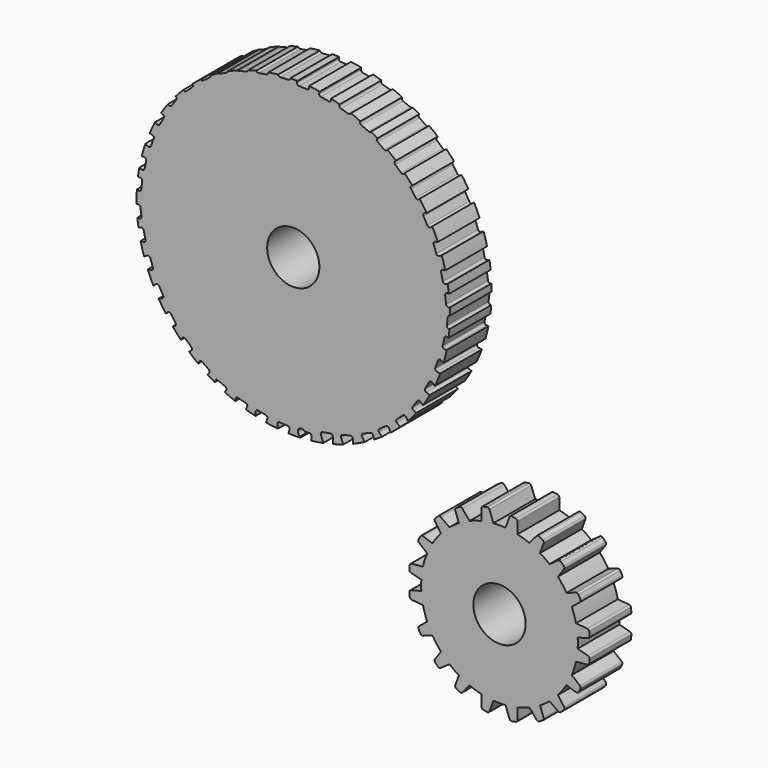
from build123d import *

# Parameters (mm, degrees)
F0_R     = 6.35
F1_DEPTH = 12.7
F2_R     = 6.35
F3_DEPTH = 6.35
F4_DEPTH = 12.7


# Not quite as in the source:
# - a feature names something its author has since deleted; it is built from what else it names


with BuildPart() as f1:
    # F0 (on Front) → F1 (new body)
    with BuildSketch(Plane.XZ):
        with BuildLine():
            ThreePointArc((10.9997188912, 27.5581906646), (10.9998077873, 27.6057086098), (10.9998374194, 27.6532266289))
            ThreePointArc((10.9998374194, 27.6532266289), (10.9910152614, 28.4730867424), (10.9645528732, 29.2925671742))
            Line((10.9645528732, 29.2925671742), (10.7348382856, 29.2197734001))
            ThreePointArc((10.7348382856, 29.2197734001), (10.3090510106, 29.2752036537), (10.0778222636, 29.6370055099))
            Line((10.0778222636, 29.6370055099), (9.8220033848, 31.5586845929))
            ThreePointArc((9.8220033848, 31.5586845929), (9.9505287127, 31.96837784), (10.3469864363, 32.1332674697))
            Line((10.3469864363, 32.1332674697), (10.7374728979, 32.1167836625))
            ThreePointArc((10.7374728979, 32.1167836625), (10.6025380467, 33.1410645829), (10.4398806598, 34.1613103339))
            Line((10.4398806598, 34.1613103339), (9.9591086943, 33.9605689489))
            ThreePointArc((9.9591086943, 33.9605689489), (9.5300858292, 33.9780817406), (9.2677308241, 34.3179893279))
            Line((9.2677308241, 34.3179893279), (8.8427687035, 36.2094704916))
            ThreePointArc((8.8427687035, 36.2094704916), (8.9345144752, 36.6289344709), (9.314815571, 36.8282793809))
            Line((9.314815571, 36.8282793809), (9.8721533535, 36.8541969291))
            ThreePointArc((9.8721533535, 36.8541969291), (9.4699352014, 38.3414420184), (9.0079175064, 39.811209703))
            Line((9.0079175064, 39.811209703), (8.4039697241, 39.4688653608))
            ThreePointArc((8.4039697241, 39.4688653608), (7.9759406786, 39.4348293087), (7.674735783, 39.7408406278))
            Line((7.674735783, 39.7408406278), (7.0261247489, 41.5677499095))
            ThreePointArc((7.0261247489, 41.5677499095), (7.0669322446, 41.9951865303), (7.4205982455, 42.2386771389))
            Line((7.4205982455, 42.2386771389), (8.0532126762, 42.3450681763))
            ThreePointArc((8.0532126762, 42.3450681763), (7.4021635025, 43.8148940816), (6.6896909802, 45.2559479055))
            Line((6.6896909802, 45.2559479055), (6.306212971, 44.9339528718))
            ThreePointArc((6.306212971, 44.9339528718), (5.8915008094, 44.8226823023), (5.539690769, 45.0688469058))
            Line((5.539690769, 45.0688469058), (4.5698129336, 46.7474268953))
            ThreePointArc((4.5698129336, 46.7474268953), (4.5322468252, 47.1751605789), (4.8357628076, 47.4788797996))
            Line((4.8357628076, 47.4788797996), (5.3257876329, 47.6574200081))
            ThreePointArc((5.3257876329, 47.6574200081), (4.5033634367, 48.9329621365), (3.63079132, 50.1747379539))
            Line((3.63079132, 50.1747379539), (3.4411244827, 49.9830087806))
            ThreePointArc((3.4411244827, 49.9830087806), (3.0384391107, 49.8339725172), (2.6654295416, 50.0466487452))
            Line((2.6654295416, 50.0466487452), (1.5449052905, 51.6286472279))
            ThreePointArc((1.5449052905, 51.6286472279), (1.4680588038, 52.0510947798), (1.742276434, 52.381506656))
            Line((1.742276434, 52.381506656), (1.8437067996, 52.4294738286))
            ThreePointArc((1.8437067996, 52.4294738286), (0.9185212718, 53.4711149077), (-0.044128746, 54.4782342364))
            Line((-0.044128746, 54.4782342364), (-0.1099293962, 54.3743183929))
            ThreePointArc((-0.1099293962, 54.3743183929), (-0.4714291441, 54.1426176184), (-0.8812897937, 54.2706081044))
            Line((-0.8812897937, 54.2706081044), (-2.3141954623, 55.5763933629))
            ThreePointArc((-2.3141954623, 55.5763933629), (-2.479602409, 55.9726355346), (-2.2823848312, 56.3540441653))
            Line((-2.2823848312, 56.3540441653), (-2.155429431, 56.4520163273))
            ThreePointArc((-2.155429431, 56.4520163274), (-3.1700394132, 57.3004727944), (-4.2134872008, 58.1132018433))
            Line((-4.2134872008, 58.1132018433), (-4.2235525545, 58.0920996826))
            ThreePointArc((-4.2235525545, 58.0920996826), (-4.5548743062, 57.8189821009), (-4.9770640288, 57.8972326901))
            Line((-4.9770640288, 57.8972326901), (-6.5553283188, 59.0230104781))
            ThreePointArc((-6.5553283188, 59.0230104781), (-6.765991691, 59.3879047844), (-6.6288005117, 59.7862833625))
            ThreePointArc((-6.6288005117, 59.7862833625), (-7.395295474, 60.2619403771), (-8.1728368701, 60.7193171364))
            ThreePointArc((-8.1728368701, 60.7193171364), (-8.4440936015, 60.5462785431), (-8.7648986851, 60.570909163))
            Line((-8.7648986851, 60.570909163), (-10.5513587328, 61.3238064301))
            ThreePointArc((-10.5513587328, 61.3238064301), (-10.8394888709, 61.6421589707), (-10.7808231589, 62.0675125305))
            Line((-10.7808231589, 62.0675125305), (-10.7740288476, 62.0780339244))
            ThreePointArc((-10.7740288476, 62.0780339244), (-11.9114103089, 62.5947750266), (-13.0651215331, 63.0739496988))
            ThreePointArc((-13.0651215331, 63.0739496988), (-13.308737144, 62.780369269), (-13.687996631, 62.7391348639))
            Line((-13.687996631, 62.7391348639), (-15.5529276076, 63.2685933129))
            ThreePointArc((-15.5529276076, 63.2685933129), (-15.8777243682, 63.5494391441), (-15.8713593131, 63.9787721183))
            Line((-15.8713593131, 63.9787721183), (-15.8367193146, 64.050271094))
            ThreePointArc((-15.8367193146, 64.050271094), (-16.8664088252, 64.3530942591), (-17.9042195936, 64.6267933027))
            Line((-17.9042195936, 64.6267933027), (-17.9048293367, 64.3664165893))
            ThreePointArc((-17.9048293367, 64.3664165893), (-18.0872040332, 63.9776920253), (-18.5022125206, 63.8675318148))
            Line((-18.5022125206, 63.8675318148), (-20.4105987179, 64.2086416483))
            ThreePointArc((-20.4105987179, 64.2086416483), (-20.7617486486, 64.4557469755), (-20.7981698105, 64.8835796713))
            Line((-20.7981698105, 64.8835796713), (-20.6791346872, 65.2082582597))
            ThreePointArc((-20.6791346872, 65.2082582597), (-21.9733949544, 65.4067198938), (-23.2737104471, 65.5605908748))
            Line((-23.2737104471, 65.5605908748), (-23.236864005, 65.2838050588))
            ThreePointArc((-23.236864005, 65.2838050588), (-23.3653893328, 64.8741118118), (-23.7618470564, 64.709222182))
            Line((-23.7618470564, 64.709222182), (-25.6987539983, 64.7909858376))
            ThreePointArc((-25.6987539983, 64.7909858376), (-26.0799048953, 64.9887010627), (-26.1734453199, 65.4077684864))
            Line((-26.1734453199, 65.4077684864), (-26.1002719199, 65.740103879))
            ThreePointArc((-26.1002719199, 65.740103879), (-26.9648411973, 65.7529863148), (-27.8294801715, 65.7462456199))
            ThreePointArc((-27.8294801715, 65.7462456199), (-27.9804758504, 65.4141090568), (-28.3151593807, 65.2688461018))
            Line((-28.3151593807, 65.2688461018), (-30.2520663226, 65.1870824461))
            ThreePointArc((-30.2520663226, 65.1870824461), (-30.579618702, 65.2892290657), (-30.767521052, 65.5763130255))
            ThreePointArc((-30.767521052, 65.5763130255), (-31.9815332506, 65.4392322445), (-33.190526184, 65.2632980351))
            ThreePointArc((-33.190526184, 65.2632980351), (-33.2795908388, 64.890932176), (-33.603314661, 64.6865019124))
            Line((-33.603314661, 64.6865019124), (-35.5117008584, 64.3453920789))
            ThreePointArc((-35.5117008584, 64.3453920789), (-35.858172076, 64.4073221349), (-36.0812348157, 64.6795732149))
            ThreePointArc((-36.0812348157, 64.6795732149), (-37.0957600333, 64.4186727919), (-38.1027291762, 64.1299798878))
            ThreePointArc((-38.1027291762, 64.1299798878), (-38.2284934828, 63.8883687789), (-38.4609857713, 63.746453577))
            Line((-38.4609857713, 63.746453577), (-40.325916748, 63.2169951281))
            ThreePointArc((-40.325916748, 63.2169951281), (-40.5089917117, 63.1996208677), (-40.6862566858, 63.2485640618))
            ThreePointArc((-40.6862566858, 63.2485640618), (-41.9303127886, 62.7484776582), (-43.1560023326, 62.2049271639))
            ThreePointArc((-43.1560023326, 62.2049271639), (-43.2554297219, 61.9623619367), (-43.4625546462, 61.8016666943))
            Line((-43.4625546462, 61.8016666943), (-45.2490146938, 61.0487694271))
            ThreePointArc((-45.2490146938, 61.0487694271), (-45.375143841, 61.0139029847), (-45.5059949449, 61.0124132943))
            ThreePointArc((-45.5059949449, 61.0124132943), (-46.3852858073, 60.5119244444), (-47.2509772507, 59.9882644073))
            ThreePointArc((-47.2509772507, 59.9882644073), (-47.2862171184, 59.7153623746), (-47.4585850602, 59.5008707422))
            Line((-47.4585850602, 59.5008707422), (-49.0368493501, 58.3750929543))
            ThreePointArc((-49.0368493501, 58.3750929543), (-49.3340936045, 58.280667011), (-49.6304916926, 58.3777163742))
            ThreePointArc((-49.6304916926, 58.3777163742), (-50.6630403611, 57.5931797134), (-51.6682920146, 56.7739583524))
            ThreePointArc((-51.6682920146, 56.7739583524), (-51.5343700759, 56.4075721833), (-51.6997179166, 56.0542536271))
            Line((-51.6997179166, 56.0542536271), (-53.1326235853, 54.7484683686))
            ThreePointArc((-53.1326235853, 54.7484683686), (-53.4988929438, 54.6165196483), (-53.8510076529, 54.7825887283))
            ThreePointArc((-53.8510076529, 54.7825887283), (-54.7920642825, 53.8213098628), (-55.6985988975, 52.8274086459))
            ThreePointArc((-55.6985988975, 52.8274086459), (-55.4746545299, 52.4968286533), (-55.5588186695, 52.1065074921))
            Line((-55.5588186695, 52.1065074921), (-56.6793429206, 50.5245090093))
            ThreePointArc((-56.6793429206, 50.5245090093), (-57.0523524897, 50.3118327813), (-57.4550378616, 50.4608690448))
            Line((-57.4550378616, 50.4608690448), (-57.5485150255, 50.5553626295))
            ThreePointArc((-57.5485150255, 50.5553626295), (-58.4221627735, 49.3452137189), (-59.2477420524, 48.1017750886))
            Line((-59.2477420524, 48.1017750886), (-58.8496761866, 47.9567400637))
            ThreePointArc((-58.8496761866, 47.9567400637), (-58.5461602041, 47.6530208431), (-58.5837263125, 47.2252871595))
            Line((-58.5837263125, 47.2252871595), (-59.5536041479, 45.5467071699))
            ThreePointArc((-59.5536041479, 45.5467071699), (-59.9054141884, 45.3005425665), (-60.32012635, 45.411813136))
            Line((-60.32012635, 45.411813136), (-60.6575622622, 45.6951479957))
            ThreePointArc((-60.6575622622, 45.6951479957), (-61.3845046078, 44.2723087866), (-62.0511517876, 42.8202419401))
            Line((-62.0511517876, 42.8202419401), (-61.4345116244, 42.716537403))
            ThreePointArc((-61.4345116244, 42.716537403), (-61.0808456236, 42.4730467945), (-61.0400381279, 42.0456101736))
            Line((-61.0400381279, 42.0456101736), (-61.688649162, 40.218700892))
            ThreePointArc((-61.688649162, 40.218700892), (-61.9898540576, 39.9126895728), (-62.417883103, 39.946725625))
            Line((-62.417883103, 39.946725625), (-63.0401527402, 40.2994556056))
            ThreePointArc((-63.0401527402, 40.2994556056), (-63.5249931039, 38.8264858378), (-63.9494927712, 37.3350066567))
            Line((-63.9494927712, 37.3350066567), (-63.32872895, 37.3061396451))
            ThreePointArc((-63.32872895, 37.3061396451), (-62.9484278542, 37.1067947351), (-62.8566820824, 36.6873307558))
            Line((-62.8566820824, 36.6873307558), (-63.2816442031, 34.795849592))
            ThreePointArc((-63.2816442031, 34.795849592), (-63.5439992082, 34.4559420048), (-63.9730220732, 34.438429213))
            Line((-63.9730220732, 34.438429213), (-64.5469466689, 34.6780655199))
            ThreePointArc((-64.5469466689, 34.6780655199), (-64.7275042773, 33.6359648683), (-64.8790671854, 32.5892540664))
            Line((-64.8790671854, 32.5892540664), (-64.3608998152, 32.6111277339))
            ThreePointArc((-64.3608998152, 32.6111277339), (-63.9644420916, 32.4462381041), (-63.8359167638, 32.0365448571))
            Line((-63.8359167638, 32.0365448571), (-64.0917356425, 30.1148657741))
            ThreePointArc((-64.0917356425, 30.1148657741), (-64.3229643895, 29.7530639179), (-64.7487516646, 29.6976336643))
            Line((-64.7487516646, 29.6976336643), (-65.1384359221, 29.8211198918))
            ThreePointArc((-65.1384359221, 29.8211198918), (-65.1957631529, 28.2322059321), (-65.186748072, 26.6422836979))
            Line((-65.186748072, 26.6422836979), (-64.9351634468, 26.7220078224))
            ThreePointArc((-64.9351634468, 26.7220078224), (-64.5093761718, 26.6665775688), (-64.2781474248, 26.3047757126))
            Line((-64.2781474248, 26.3047757126), (-64.022328546, 24.3830966296))
            ThreePointArc((-64.022328546, 24.3830966296), (-64.1508538739, 23.9734033826), (-64.5473115975, 23.8085137528))
            Line((-64.5473115975, 23.8085137528), (-65.0076450673, 23.8279460479))
            ThreePointArc((-65.0076450673, 23.8279460479), (-64.8874574844, 22.7818465517), (-64.7384071979, 21.7394679146))
            Line((-64.7384071979, 21.7394679146), (-64.1594338555, 21.9812122737))
            ThreePointArc((-64.1594338555, 21.9812122737), (-63.7304109905, 21.9636994819), (-63.4680559853, 21.6237918947))
            Line((-63.4680559853, 21.6237918947), (-63.0430938647, 19.732310731))
            ThreePointArc((-63.0430938647, 19.732310731), (-63.1348396364, 19.3128467516), (-63.5151407322, 19.1135018416))
            Line((-63.5151407322, 19.1135018416), (-64.22319658, 19.0805755407))
            ThreePointArc((-64.22319658, 19.0805755407), (-63.8353518953, 17.546997559), (-63.3841831012, 16.0308406922))
            Line((-63.3841831012, 16.0308406922), (-62.6042948853, 16.4729158617))
            ThreePointArc((-62.6042948853, 16.4729158617), (-62.1762658398, 16.5069519139), (-61.8750609442, 16.2009405947))
            Line((-61.8750609442, 16.2009405947), (-61.2264499102, 14.3740313131))
            ThreePointArc((-61.2264499102, 14.3740313131), (-61.2672574059, 13.9465946922), (-61.6209234067, 13.7031040837))
            Line((-61.6209234067, 13.7031040837), (-62.496147031, 13.5559118211))
            ThreePointArc((-62.496147031, 13.5559118211), (-61.840661676, 12.0100900315), (-61.1177054988, 10.4946493624))
            Line((-61.1177054988, 10.4946493624), (-60.5065381322, 11.0078283507))
            ThreePointArc((-60.5065381322, 11.0078283507), (-60.0918259707, 11.1190989202), (-59.7400159302, 10.8729343168))
            Line((-59.7400159302, 10.8729343168), (-58.7701380948, 9.1943543272))
            ThreePointArc((-58.7701380948, 9.1943543272), (-58.7325719864, 8.7666206436), (-59.0360879688, 8.462901423))
            Line((-59.0360879688, 8.462901423), (-59.8414658167, 8.1694625572))
            ThreePointArc((-59.8414658167, 8.1694625572), (-58.9970313158, 6.8157660137), (-58.0966620118, 5.4986103377))
            Line((-58.0966620118, 5.4986103377), (-57.6414496439, 5.9587724419))
            ThreePointArc((-57.6414496439, 5.9587724419), (-57.2387642719, 6.1078087054), (-56.8657547028, 5.8951324774))
            Line((-56.8657547028, 5.8951324774), (-55.7452304518, 4.3131339946))
            ThreePointArc((-55.7452304518, 4.3131339946), (-55.6683839651, 3.8906864428), (-55.9426015952, 3.5602745666))
            Line((-55.9426015952, 3.5602745666), (-56.4268233767, 3.331282493))
            ThreePointArc((-56.4268233767, 3.331282493), (-55.4362444187, 2.1840989237), (-54.4008215813, 1.0772220735))
            Line((-54.4008215813, 1.0772220735), (-54.090395765, 1.5674628297))
            ThreePointArc((-54.090395765, 1.5674628297), (-53.7288960171, 1.7991636042), (-53.3190353676, 1.6711731181))
            Line((-53.3190353676, 1.6711731181), (-51.8861296989, 0.3653878596))
            ThreePointArc((-51.8861296989, 0.3653878596), (-51.7207227522, -0.030854312), (-51.9179403301, -0.4122629427))
            Line((-51.9179403301, -0.4122629427), (-52.430008547, -0.8074287276))
            ThreePointArc((-52.430008547, -0.8074287276), (-51.3370345705, -1.7437806362), (-50.209476255, -2.63818505))
            Line((-50.209476255, -2.63818505), (-49.9767726067, -2.15031846))
            ThreePointArc((-49.9767726067, -2.15031846), (-49.645450855, -1.8772008783), (-49.2232611324, -1.9554514676))
            Line((-49.2232611324, -1.9554514676), (-47.6449968424, -3.0812292555))
            ThreePointArc((-47.6449968424, -3.0812292555), (-47.4335619489, -3.4549438557), (-47.5839362118, -3.8571314955))
            Line((-47.5839362118, -3.8571314955), (-47.9614222989, -4.2280820483))
            ThreePointArc((-47.9614222989, -4.2280820482), (-47.0894340376, -4.7819244671), (-46.2027512987, -5.3119232156))
            Line((-46.2027512987, -5.3119232156), (-46.1279879303, -4.9842494954))
            ThreePointArc((-46.1279879303, -4.9842494954), (-45.8645051535, -4.645215363), (-45.4354264761, -4.6291279404))
            Line((-45.4354264761, -4.6291279404), (-43.6489664284, -5.3820252075))
            ThreePointArc((-43.6489664284, -5.3820252075), (-43.3608362903, -5.7003777482), (-43.4195020023, -6.1257313079))
            Line((-43.4195020023, -6.1257313079), (-43.7395109331, -6.6212841102))
            ThreePointArc((-43.7395109331, -6.6212841102), (-42.4839429692, -7.2028962329), (-41.2080832693, -7.7385319293))
            Line((-41.2080832693, -7.7385319293), (-41.1564230384, -7.2342689091))
            ThreePointArc((-41.1564230384, -7.2342689091), (-40.936244252, -6.8656381744), (-40.5123285302, -6.7973536414))
            Line((-40.5123285302, -6.7973536414), (-38.6473975536, -7.3268120903))
            ThreePointArc((-38.6473975536, -7.3268120903), (-38.3226007931, -7.6076579216), (-38.3289658481, -8.0369908957))
            Line((-38.3289658481, -8.0369908957), (-38.6308254122, -8.6600466285))
            ThreePointArc((-38.6308254122, -8.6600466285), (-37.4694601461, -9.0085745816), (-36.2975924953, -9.3199701894))
            Line((-36.2975924953, -9.3199701894), (-36.2954958245, -8.4246353667))
            ThreePointArc((-36.2954958245, -8.4246353667), (-36.113121128, -8.0359108027), (-35.6981126406, -7.9257505922))
            Line((-35.6981126406, -7.9257505922), (-33.7897264433, -8.2668604257))
            ThreePointArc((-33.7897264433, -8.2668604257), (-33.4385765126, -8.5139657529), (-33.4021553507, -8.9417984487))
            Line((-33.4021553507, -8.9417984487), (-33.7401508156, -9.8637102962))
            ThreePointArc((-33.7401508156, -9.8637102962), (-32.2943574101, -10.0910489645), (-30.8408994302, -10.262692031))
            Line((-30.8408994302, -10.262692031), (-30.9634611563, -9.3420238363))
            ThreePointArc((-30.9634611563, -9.3420238363), (-30.8349358284, -8.9323305892), (-30.4384781048, -8.7674409594))
            Line((-30.4384781048, -8.7674409594), (-28.501571163, -8.8492046151))
            ThreePointArc((-28.501571163, -8.8492046151), (-28.1204202659, -9.0469198402), (-28.0268798413, -9.4659872638))
            Line((-28.0268798413, -9.4659872638), (-28.239079823, -10.4297468306))
            ThreePointArc((-28.239079823, -10.4297468306), (-26.7997598376, -10.445589077), (-25.3608686191, -10.4070526201))
            Line((-25.3608686191, -10.4070526201), (-25.4212528924, -10.1328022615))
            ThreePointArc((-25.4212528924, -10.1328022615), (-25.9545068406, -9.5738274901), (-25.8690763539, -8.8060292092))
            Line((-25.8690763539, -8.8060292092), (-25.714814749, -8.7995172842))
            Line((-25.714814749, -8.7995172842), (-25.7480149898, -8.6487300437))
            ThreePointArc((-25.7480149898, -8.6487300437), (-25.0276801925, -8.3695699677), (-24.350808885, -8.7419377984))
            Line((-24.350808885, -8.7419377984), (-23.1730356776, -8.6922198482))
            ThreePointArc((-23.1730356776, -8.6922198482), (-22.776577954, -8.8571094779), (-22.6480526262, -9.266802725))
            Line((-22.6480526262, -9.266802725), (-22.7723049069, -10.2001701534))
            ThreePointArc((-22.7723049069, -10.2001701534), (-21.2829449331, -10.0000597993), (-19.802634675, -9.7413730677))
            Line((-19.802634675, -9.7413730677), (-20.3937118727, -8.1291589168))
            ThreePointArc((-20.3937118727, -8.1291589168), (-20.3572907108, -7.7013262211), (-20.0061407801, -7.4542208939))
            Line((-20.0061407801, -7.4542208939), (-18.0977545828, -7.1131110603))
            ThreePointArc((-18.0977545828, -7.1131110603), (-17.6827460954, -7.2232712708), (-17.5003713989, -7.6119958349))
            Line((-17.5003713989, -7.6119958349), (-17.4966138523, -9.2165692998))
            ThreePointArc((-17.4966138523, -9.2165692998), (-16.1816895504, -8.8487862839), (-14.8807877497, -8.4341240461))
            Line((-14.8807877497, -8.4341240461), (-15.4669013753, -7.2243513638))
            ThreePointArc((-15.4669013753, -7.2243513638), (-15.4732664304, -6.7950183897), (-15.1484696698, -6.5141725585))
            Line((-15.1484696698, -6.5141725585), (-13.2835386932, -5.9847141095))
            ThreePointArc((-13.2835386932, -5.9847141095), (-12.8596229715, -6.0529986425), (-12.639444185, -6.4216293772))
            Line((-12.639444185, -6.4216293772), (-12.5240221267, -7.5482808597))
            ThreePointArc((-12.5240221267, -7.5482808597), (-11.1281345097, -6.9372969188), (-9.757793639, -6.2709865454))
            Line((-9.757793639, -6.2709865454), (-10.3763652211, -5.3130917761))
            ThreePointArc((-10.3763652211, -5.3130917761), (-10.4350309331, -4.8877382163), (-10.146900795, -4.5693856757))
            Line((-10.146900795, -4.5693856757), (-8.3604407473, -3.8164884085))
            ThreePointArc((-8.3604407473, -3.8164884085), (-7.9313620699, -3.8325758311), (-7.6678792931, -4.1716099635))
            Line((-7.6678792931, -4.1716099635), (-7.4776978111, -5.0051394718))
            ThreePointArc((-7.4776978111, -5.0051394718), (-6.4826678485, -4.3862632386), (-5.5071401804, -3.7370805315))
            Line((-5.5071401804, -3.7370805315), (-6.2119310116, -3.0444919636))
            ThreePointArc((-6.2119310116, -3.0444919636), (-6.3623052745, -2.6423043238), (-6.150870381, -2.2685897236))
            Line((-6.150870381, -2.2685897236), (-4.572606091, -1.1428119357))
            ThreePointArc((-4.572606091, -1.1428119357), (-4.1504163684, -1.0645613464), (-3.8190946167, -1.3376789282))
            Line((-3.8190946167, -1.3376789282), (-3.4131963694, -2.188650519))
            ThreePointArc((-3.4131963694, -2.188650519), (-2.2377168726, -1.2166329727), (-1.102085699, -0.1983442147))
            Line((-1.102085699, -0.1983442147), (-1.8779268934, 0.4003765891))
            ThreePointArc((-1.8779268934, 0.4003765891), (-2.0751444712, 0.7817852198), (-1.9097375245, 1.1780273915))
            Line((-1.9097375245, 1.1780273915), (-0.4768318558, 2.48381265))
            ThreePointArc((-0.4768318558, 2.48381265), (-0.0669712063, 2.611803136), (0.2945285416, 2.3801023615))
            Line((0.2945285416, 2.3801023615), (0.7527001057, 1.6565337589))
            ThreePointArc((0.7527001057, 1.6565337589), (1.8082121295, 2.8355742094), (2.81385293, 4.057428782))
            Line((2.81385293, 4.057428782), (2.1467343718, 4.3729140985))
            ThreePointArc((2.1467343718, 4.3729140985), (1.8725167416, 4.7033259747), (1.9493632283, 5.1257735265))
            Line((1.9493632283, 5.1257735265), (3.0698874794, 6.7077720093))
            ThreePointArc((3.0698874794, 6.7077720093), (3.4428970485, 6.9204482372), (3.8455824205, 6.7714119738))
            Line((3.8455824205, 6.7714119738), (4.3960431351, 6.2149658432))
            ThreePointArc((4.3960431351, 6.2149658432), (5.2772221083, 7.570523606), (6.1000969144, 8.9622456632))
            Line((6.1000969144, 8.9622456632), (5.2402207454, 9.2755409549))
            ThreePointArc((5.2402207454, 9.2755409549), (4.936704763, 9.5792601755), (4.9742708714, 10.0069938591))
            Line((4.9742708714, 10.0069938591), (5.9441487068, 11.6855738486))
            ThreePointArc((5.9441487068, 11.6855738486), (6.2959587472, 11.9317384521), (6.7106709088, 11.8204678826))
            Line((6.7106709088, 11.8204678826), (7.3171250079, 11.3112464842))
            ThreePointArc((7.3171250079, 11.3112464842), (7.9992572968, 12.8329457858), (8.6141490481, 14.383036544))
            Line((8.6141490481, 14.383036544), (7.8250561833, 14.5157436156))
            ThreePointArc((7.8250561833, 14.5157436156), (7.4713901824, 14.7592342241), (7.4305826868, 15.186670845))
            Line((7.4305826868, 15.186670845), (8.0791937208, 17.0135801266))
            ThreePointArc((8.0791937208, 17.0135801266), (8.3803986164, 17.3195914457), (8.8084276619, 17.2855553936))
            Line((8.8084276619, 17.2855553936), (9.4562609049, 16.9183348293))
            ThreePointArc((9.4562609049, 16.9183348293), (9.8599696449, 18.4034360436), (10.2033727185, 19.9036295952))
            Line((10.2033727185, 19.9036295952), (9.7192735088, 19.9261413735))
            ThreePointArc((9.7192735088, 19.9261413735), (9.338972413, 20.1254862835), (9.2472266413, 20.5449502628))
            Line((9.2472266413, 20.5449502628), (9.6721887619, 22.4364314266))
            ThreePointArc((9.6721887619, 22.4364314266), (9.934543767, 22.7763390138), (10.3635666321, 22.7938518055))
            Line((10.3635666321, 22.7938518055), (10.6718998082, 22.6651104619))
            ThreePointArc((10.6718998082, 22.6651104619), (10.7883585152, 23.6444900236), (10.8794275214, 24.6265559036))
            Line((10.8794275214, 24.6265559036), (10.7514443741, 24.6211532847))
            ThreePointArc((10.7514443741, 24.6211532847), (10.3549866505, 24.7860429144), (10.2264613226, 25.1957361615))
            Line((10.2264613226, 25.1957361615), (10.4822802014, 27.1174152445))
            ThreePointArc((10.4822802014, 27.1174152445), (10.6564193702, 27.4370940073), (10.9997188912, 27.5581906646))
        make_face()
        with Locations((-27.1001625806, 27.6532266289)):
            Circle(F0_R, mode=Mode.SUBTRACT)
    extrude(amount=F1_DEPTH)


with BuildPart() as f3:
    # F2 (on Front) → F3 (new body)
    with BuildSketch(Plane.XZ):
        with BuildLine():
            ThreePointArc((42.0565411949, -33.6461532038), (42.0848993622, -33.0466002404), (42.0943552136, -32.4464514852))
            ThreePointArc((42.0943552136, -32.4464514852), (42.0848993622, -31.8463027299), (42.0565411949, -31.2467497665))
            Line((42.0565411949, -31.2467497665), (41.9391885765, -31.2781943059))
            ThreePointArc((41.9391885765, -31.2781943059), (41.5163316719, -31.2036332246), (41.3016415949, -30.8317791034))
            Line((41.3016415949, -30.8317791034), (41.1326786883, -28.9005242438))
            ThreePointArc((41.1326786883, -28.9005242438), (41.2674640116, -28.5095302405), (41.6483327178, -28.3483396))
            ThreePointArc((41.6483327178, -28.3483396), (41.2128175391, -26.7184957653), (40.6348161174, -25.1335734476))
            Line((40.6348161174, -25.1335734476), (40.4924962803, -25.2502185345))
            ThreePointArc((40.4924962803, -25.2502185345), (40.0764905603, -25.3565508322), (39.7276319722, -25.1062210455))
            Line((39.7276319722, -25.1062210455), (38.7777788943, -23.4162290553))
            ThreePointArc((38.7777788943, -23.4162290553), (38.7453006584, -22.9880789872), (39.0524060312, -22.6879896562))
            Line((39.0524060312, -22.6879896562), (39.3437173132, -22.5857570295))
            ThreePointArc((39.3437173132, -22.5857570295), (38.3744958595, -21.1376368798), (37.277005557, -19.7841387342))
            Line((37.277005557, -19.7841387342), (37.1709426873, -19.9356122101))
            ThreePointArc((37.1709426873, -19.9356122101), (36.7990885661, -20.1503022871), (36.3956032039, -20.0034456253))
            Line((36.3956032039, -20.0034456253), (35.0247834133, -18.6326258346))
            ThreePointArc((35.0247834133, -18.6326258346), (34.8779267515, -18.2291404725), (35.0926168285, -17.8572863513))
            Line((35.0926168285, -17.8572863513), (35.2022178765, -17.7805428713))
            ThreePointArc((35.2022178765, -17.7805428713), (34.0889353894, -16.9248617231), (32.9156495595, -16.1535067563))
            Line((32.9156495595, -16.1535067563), (32.852178634, -16.3278916908))
            ThreePointArc((32.852178634, -16.3278916908), (32.5485610154, -16.6315093094), (32.1208147826, -16.5940863631))
            Line((32.1208147826, -16.5940863631), (30.4419102744, -15.6247703934))
            ThreePointArc((30.4419102744, -15.6247703934), (30.1956279359, -15.2730427625), (30.3067596973, -14.8582933825))
            Line((30.3067596973, -14.8582933825), (30.3212189182, -14.8410615541))
            ThreePointArc((30.3212189182, -14.8410615541), (28.894842847, -14.3170749252), (27.4312407343, -13.9084436249))
            Line((27.4312407343, -13.9084436249), (27.4312407343, -13.921173552))
            ThreePointArc((27.4312407343, -13.921173552), (27.2497768401, -14.3103241291), (26.8350274601, -14.4214558905))
            Line((26.8350274601, -14.4214558905), (24.9258476959, -14.084815987))
            ThreePointArc((24.9258476959, -14.084815987), (24.5858631842, -13.8578661496), (24.5231355059, -13.4539343048))
            ThreePointArc((24.5231355059, -13.4539343048), (23.0443552136, -13.3964514852), (21.5655749214, -13.4539343048))
            ThreePointArc((21.5655749214, -13.4539343048), (21.5028472431, -13.8578661496), (21.1628627314, -14.084815987))
            Line((21.1628627314, -14.084815987), (19.2536829672, -14.4214558905))
            ThreePointArc((19.2536829672, -14.4214558905), (18.8389335872, -14.3103241291), (18.6574696929, -13.921173552))
            Line((18.6574696929, -13.921173552), (18.6574696929, -13.9084436249))
            ThreePointArc((18.6574696929, -13.9084436249), (17.1938675803, -14.3170749252), (15.7674915091, -14.8410615541))
            Line((15.7674915091, -14.8410615541), (15.7819507299, -14.8582933825))
            ThreePointArc((15.7819507299, -14.8582933825), (15.8930824914, -15.2730427625), (15.6468001528, -15.6247703934))
            Line((15.6468001528, -15.6247703934), (13.9678956447, -16.5940863631))
            ThreePointArc((13.9678956447, -16.5940863631), (13.5401494119, -16.6315093094), (13.2365317933, -16.3278916908))
            Line((13.2365317933, -16.3278916908), (13.1730608678, -16.1535067563))
            ThreePointArc((13.1730608678, -16.1535067563), (11.9997750379, -16.9248617231), (10.8864925508, -17.7805428713))
            Line((10.8864925508, -17.7805428713), (10.9960935988, -17.8572863513))
            ThreePointArc((10.9960935988, -17.8572863513), (11.2107836758, -18.2291404725), (11.063927014, -18.6326258346))
            Line((11.063927014, -18.6326258346), (9.6931072233, -20.0034456253))
            ThreePointArc((9.6931072233, -20.0034456253), (9.2896218612, -20.1503022871), (8.91776774, -19.9356122101))
            Line((8.91776774, -19.9356122101), (8.8117048703, -19.7841387342))
            ThreePointArc((8.8117048703, -19.7841387342), (7.7142145678, -21.1376368798), (6.7449931141, -22.5857570295))
            Line((6.7449931141, -22.5857570295), (7.0363043961, -22.6879896562))
            ThreePointArc((7.0363043961, -22.6879896562), (7.3434097689, -22.9880789872), (7.310931533, -23.4162290553))
            Line((7.310931533, -23.4162290553), (6.3610784551, -25.1062210455))
            ThreePointArc((6.3610784551, -25.1062210455), (6.012219867, -25.3565508322), (5.596214147, -25.2502185345))
            Line((5.596214147, -25.2502185345), (5.4538943099, -25.1335734476))
            ThreePointArc((5.4538943099, -25.1335734476), (4.8758928882, -26.7184957653), (4.4403777094, -28.3483396))
            ThreePointArc((4.4403777094, -28.3483396), (4.8212464157, -28.5095302405), (4.956031739, -28.9005242438))
            Line((4.956031739, -28.9005242438), (4.7870688324, -30.8317791034))
            ThreePointArc((4.7870688324, -30.8317791034), (4.5723787554, -31.2036332246), (4.1495218508, -31.2781943059))
            Line((4.1495218508, -31.2781943059), (4.0321692324, -31.2467497665))
            ThreePointArc((4.0321692324, -31.2467497665), (3.9943552136, -32.4464514852), (4.0321692324, -33.6461532038))
            Line((4.0321692324, -33.6461532038), (4.1495218508, -33.6147086644))
            ThreePointArc((4.1495218508, -33.6147086644), (4.5723787554, -33.6892697457), (4.7870688324, -34.0611238669))
            Line((4.7870688324, -34.0611238669), (4.956031739, -35.9923787265))
            ThreePointArc((4.956031739, -35.9923787265), (4.8212464157, -36.3833727298), (4.4403777094, -36.5445633703))
            ThreePointArc((4.4403777094, -36.5445633703), (4.8758928882, -38.174407205), (5.4538943099, -39.7593295227))
            Line((5.4538943099, -39.7593295227), (5.596214147, -39.6426844358))
            ThreePointArc((5.596214147, -39.6426844358), (6.012219867, -39.5363521381), (6.3610784551, -39.7866819248))
            Line((6.3610784551, -39.7866819248), (7.310931533, -41.4766739151))
            ThreePointArc((7.310931533, -41.4766739151), (7.3434097689, -41.9048239831), (7.0363043961, -42.2049133141))
            Line((7.0363043961, -42.2049133141), (6.7449931141, -42.3071459408))
            ThreePointArc((6.7449931141, -42.3071459408), (7.7142145678, -43.7552660905), (8.8117048703, -45.1087642362))
            Line((8.8117048703, -45.1087642362), (8.91776774, -44.9572907602))
            ThreePointArc((8.91776774, -44.9572907602), (9.2896218612, -44.7426006832), (9.6931072233, -44.889457345))
            Line((9.6931072233, -44.889457345), (11.063927014, -46.2602771357))
            ThreePointArc((11.063927014, -46.2602771357), (11.2107836758, -46.6637624978), (10.9960935988, -47.035616619))
            Line((10.9960935988, -47.035616619), (10.8864925508, -47.112360099))
            ThreePointArc((10.8864925508, -47.112360099), (11.9997750379, -47.9680412472), (13.1730608678, -48.739396214))
            Line((13.1730608678, -48.739396214), (13.2365317933, -48.5650112795))
            ThreePointArc((13.2365317933, -48.5650112795), (13.5401494119, -48.261393661), (13.9678956447, -48.2988166072))
            Line((13.9678956447, -48.2988166072), (15.6468001528, -49.2681325769))
            ThreePointArc((15.6468001528, -49.2681325769), (15.8930824914, -49.6198602078), (15.7819507299, -50.0346095878))
            Line((15.7819507299, -50.0346095878), (15.7674915091, -50.0518414162))
            ThreePointArc((15.7674915091, -50.0518414162), (17.1938675803, -50.5758280451), (18.6574696929, -50.9844593455))
            Line((18.6574696929, -50.9844593455), (18.6574696929, -50.9717294183))
            ThreePointArc((18.6574696929, -50.9717294183), (18.8389335872, -50.5825788412), (19.2536829672, -50.4714470798))
            Line((19.2536829672, -50.4714470798), (21.1628627314, -50.8080869833))
            ThreePointArc((21.1628627314, -50.8080869833), (21.5028472431, -51.0350368207), (21.5655749214, -51.4389686655))
            ThreePointArc((21.5655749214, -51.4389686655), (23.0443552136, -51.4964514852), (24.5231355059, -51.4389686655))
            ThreePointArc((24.5231355059, -51.4389686655), (24.5858631842, -51.0350368207), (24.9258476959, -50.8080869833))
            Line((24.9258476959, -50.8080869833), (26.8350274601, -50.4714470798))
            ThreePointArc((26.8350274601, -50.4714470798), (27.2497768401, -50.5825788412), (27.4312407343, -50.9717294183))
            Line((27.4312407343, -50.9717294183), (27.4312407343, -50.9844593455))
            ThreePointArc((27.4312407343, -50.9844593455), (28.894842847, -50.5758280451), (30.3212189182, -50.0518414162))
            Line((30.3212189182, -50.0518414162), (30.3067596973, -50.0346095878))
            ThreePointArc((30.3067596973, -50.0346095878), (30.1956279359, -49.6198602078), (30.4419102744, -49.2681325769))
            Line((30.4419102744, -49.2681325769), (32.1208147826, -48.2988166072))
            ThreePointArc((32.1208147826, -48.2988166072), (32.5485610154, -48.261393661), (32.852178634, -48.5650112795))
            Line((32.852178634, -48.5650112795), (32.9156495595, -48.739396214))
            ThreePointArc((32.9156495595, -48.739396214), (34.0889353894, -47.9680412472), (35.2022178765, -47.112360099))
            Line((35.2022178765, -47.112360099), (35.0926168285, -47.035616619))
            ThreePointArc((35.0926168285, -47.035616619), (34.8779267515, -46.6637624978), (35.0247834133, -46.2602771357))
            Line((35.0247834133, -46.2602771357), (36.3956032039, -44.889457345))
            ThreePointArc((36.3956032039, -44.889457345), (36.7990885661, -44.7426006832), (37.1709426873, -44.9572907602))
            Line((37.1709426873, -44.9572907602), (37.277005557, -45.1087642362))
            ThreePointArc((37.277005557, -45.1087642362), (38.3744958595, -43.7552660905), (39.3437173132, -42.3071459408))
            Line((39.3437173132, -42.3071459408), (39.0524060312, -42.2049133141))
            ThreePointArc((39.0524060312, -42.2049133141), (38.7453006584, -41.9048239831), (38.7777788943, -41.4766739151))
            Line((38.7777788943, -41.4766739151), (39.7276319722, -39.7866819248))
            ThreePointArc((39.7276319722, -39.7866819248), (40.0764905603, -39.5363521381), (40.4924962803, -39.6426844358))
            Line((40.4924962803, -39.6426844358), (40.6348161174, -39.7593295227))
            ThreePointArc((40.6348161174, -39.7593295227), (41.2128175391, -38.174407205), (41.6483327178, -36.5445633703))
            ThreePointArc((41.6483327178, -36.5445633703), (41.2674640116, -36.3833727298), (41.1326786883, -35.9923787265))
            Line((41.1326786883, -35.9923787265), (41.3016415949, -34.0611238669))
            ThreePointArc((41.3016415949, -34.0611238669), (41.5163316719, -33.6892697457), (41.9391885765, -33.6147086644))
            Line((41.9391885765, -33.6147086644), (42.0565411949, -33.6461532038))
        make_face()
        with Locations((23.0443552136, -32.4464514852)):
            Circle(F2_R, mode=Mode.SUBTRACT)
    extrude(amount=F3_DEPTH)

    # F2 (on Front) → F4 (join)
    with BuildSketch(Plane.XZ):
        with BuildLine():
            ThreePointArc((42.0565411949, -33.6461532038), (42.0848993622, -33.0466002404), (42.0943552136, -32.4464514852))
            ThreePointArc((42.0943552136, -32.4464514852), (42.0848993622, -31.8463027299), (42.0565411949, -31.2467497665))
            Line((42.0565411949, -31.2467497665), (41.9391885765, -31.2781943059))
            ThreePointArc((41.9391885765, -31.2781943059), (41.5163316719, -31.2036332246), (41.3016415949, -30.8317791034))
            Line((41.3016415949, -30.8317791034), (41.1326786883, -28.9005242438))
            ThreePointArc((41.1326786883, -28.9005242438), (41.2674640116, -28.5095302405), (41.6483327178, -28.3483396))
            ThreePointArc((41.6483327178, -28.3483396), (41.2128175391, -26.7184957653), (40.6348161174, -25.1335734476))
            Line((40.6348161174, -25.1335734476), (40.4924962803, -25.2502185345))
            ThreePointArc((40.4924962803, -25.2502185345), (40.0764905603, -25.3565508322), (39.7276319722, -25.1062210455))
            Line((39.7276319722, -25.1062210455), (38.7777788943, -23.4162290553))
            ThreePointArc((38.7777788943, -23.4162290553), (38.7453006584, -22.9880789872), (39.0524060312, -22.6879896562))
            Line((39.0524060312, -22.6879896562), (39.3437173132, -22.5857570295))
            ThreePointArc((39.3437173132, -22.5857570295), (38.3744958595, -21.1376368798), (37.277005557, -19.7841387342))
            Line((37.277005557, -19.7841387342), (37.1709426873, -19.9356122101))
            ThreePointArc((37.1709426873, -19.9356122101), (36.7990885661, -20.1503022871), (36.3956032039, -20.0034456253))
            Line((36.3956032039, -20.0034456253), (35.0247834133, -18.6326258346))
            ThreePointArc((35.0247834133, -18.6326258346), (34.8779267515, -18.2291404725), (35.0926168285, -17.8572863513))
            Line((35.0926168285, -17.8572863513), (35.2022178765, -17.7805428713))
            ThreePointArc((35.2022178765, -17.7805428713), (34.0889353894, -16.9248617231), (32.9156495595, -16.1535067563))
            Line((32.9156495595, -16.1535067563), (32.852178634, -16.3278916908))
            ThreePointArc((32.852178634, -16.3278916908), (32.5485610154, -16.6315093094), (32.1208147826, -16.5940863631))
            Line((32.1208147826, -16.5940863631), (30.4419102744, -15.6247703934))
            ThreePointArc((30.4419102744, -15.6247703934), (30.1956279359, -15.2730427625), (30.3067596973, -14.8582933825))
            Line((30.3067596973, -14.8582933825), (30.3212189182, -14.8410615541))
            ThreePointArc((30.3212189182, -14.8410615541), (28.894842847, -14.3170749252), (27.4312407343, -13.9084436249))
            Line((27.4312407343, -13.9084436249), (27.4312407343, -13.921173552))
            ThreePointArc((27.4312407343, -13.921173552), (27.2497768401, -14.3103241291), (26.8350274601, -14.4214558905))
            Line((26.8350274601, -14.4214558905), (24.9258476959, -14.084815987))
            ThreePointArc((24.9258476959, -14.084815987), (24.5858631842, -13.8578661496), (24.5231355059, -13.4539343048))
            ThreePointArc((24.5231355059, -13.4539343048), (23.0443552136, -13.3964514852), (21.5655749214, -13.4539343048))
            ThreePointArc((21.5655749214, -13.4539343048), (21.5028472431, -13.8578661496), (21.1628627314, -14.084815987))
            Line((21.1628627314, -14.084815987), (19.2536829672, -14.4214558905))
            ThreePointArc((19.2536829672, -14.4214558905), (18.8389335872, -14.3103241291), (18.6574696929, -13.921173552))
            Line((18.6574696929, -13.921173552), (18.6574696929, -13.9084436249))
            ThreePointArc((18.6574696929, -13.9084436249), (17.1938675803, -14.3170749252), (15.7674915091, -14.8410615541))
            Line((15.7674915091, -14.8410615541), (15.7819507299, -14.8582933825))
            ThreePointArc((15.7819507299, -14.8582933825), (15.8930824914, -15.2730427625), (15.6468001528, -15.6247703934))
            Line((15.6468001528, -15.6247703934), (13.9678956447, -16.5940863631))
            ThreePointArc((13.9678956447, -16.5940863631), (13.5401494119, -16.6315093094), (13.2365317933, -16.3278916908))
            Line((13.2365317933, -16.3278916908), (13.1730608678, -16.1535067563))
            ThreePointArc((13.1730608678, -16.1535067563), (11.9997750379, -16.9248617231), (10.8864925508, -17.7805428713))
            Line((10.8864925508, -17.7805428713), (10.9960935988, -17.8572863513))
            ThreePointArc((10.9960935988, -17.8572863513), (11.2107836758, -18.2291404725), (11.063927014, -18.6326258346))
            Line((11.063927014, -18.6326258346), (9.6931072233, -20.0034456253))
            ThreePointArc((9.6931072233, -20.0034456253), (9.2896218612, -20.1503022871), (8.91776774, -19.9356122101))
            Line((8.91776774, -19.9356122101), (8.8117048703, -19.7841387342))
            ThreePointArc((8.8117048703, -19.7841387342), (7.7142145678, -21.1376368798), (6.7449931141, -22.5857570295))
            Line((6.7449931141, -22.5857570295), (7.0363043961, -22.6879896562))
            ThreePointArc((7.0363043961, -22.6879896562), (7.3434097689, -22.9880789872), (7.310931533, -23.4162290553))
            Line((7.310931533, -23.4162290553), (6.3610784551, -25.1062210455))
            ThreePointArc((6.3610784551, -25.1062210455), (6.012219867, -25.3565508322), (5.596214147, -25.2502185345))
            Line((5.596214147, -25.2502185345), (5.4538943099, -25.1335734476))
            ThreePointArc((5.4538943099, -25.1335734476), (4.8758928882, -26.7184957653), (4.4403777094, -28.3483396))
            ThreePointArc((4.4403777094, -28.3483396), (4.8212464157, -28.5095302405), (4.956031739, -28.9005242438))
            Line((4.956031739, -28.9005242438), (4.7870688324, -30.8317791034))
            ThreePointArc((4.7870688324, -30.8317791034), (4.5723787554, -31.2036332246), (4.1495218508, -31.2781943059))
            Line((4.1495218508, -31.2781943059), (4.0321692324, -31.2467497665))
            ThreePointArc((4.0321692324, -31.2467497665), (3.9943552136, -32.4464514852), (4.0321692324, -33.6461532038))
            Line((4.0321692324, -33.6461532038), (4.1495218508, -33.6147086644))
            ThreePointArc((4.1495218508, -33.6147086644), (4.5723787554, -33.6892697457), (4.7870688324, -34.0611238669))
            Line((4.7870688324, -34.0611238669), (4.956031739, -35.9923787265))
            ThreePointArc((4.956031739, -35.9923787265), (4.8212464157, -36.3833727298), (4.4403777094, -36.5445633703))
            ThreePointArc((4.4403777094, -36.5445633703), (4.8758928882, -38.174407205), (5.4538943099, -39.7593295227))
            Line((5.4538943099, -39.7593295227), (5.596214147, -39.6426844358))
            ThreePointArc((5.596214147, -39.6426844358), (6.012219867, -39.5363521381), (6.3610784551, -39.7866819248))
            Line((6.3610784551, -39.7866819248), (7.310931533, -41.4766739151))
            ThreePointArc((7.310931533, -41.4766739151), (7.3434097689, -41.9048239831), (7.0363043961, -42.2049133141))
            Line((7.0363043961, -42.2049133141), (6.7449931141, -42.3071459408))
            ThreePointArc((6.7449931141, -42.3071459408), (7.7142145678, -43.7552660905), (8.8117048703, -45.1087642362))
            Line((8.8117048703, -45.1087642362), (8.91776774, -44.9572907602))
            ThreePointArc((8.91776774, -44.9572907602), (9.2896218612, -44.7426006832), (9.6931072233, -44.889457345))
            Line((9.6931072233, -44.889457345), (11.063927014, -46.2602771357))
            ThreePointArc((11.063927014, -46.2602771357), (11.2107836758, -46.6637624978), (10.9960935988, -47.035616619))
            Line((10.9960935988, -47.035616619), (10.8864925508, -47.112360099))
            ThreePointArc((10.8864925508, -47.112360099), (11.9997750379, -47.9680412472), (13.1730608678, -48.739396214))
            Line((13.1730608678, -48.739396214), (13.2365317933, -48.5650112795))
            ThreePointArc((13.2365317933, -48.5650112795), (13.5401494119, -48.261393661), (13.9678956447, -48.2988166072))
            Line((13.9678956447, -48.2988166072), (15.6468001528, -49.2681325769))
            ThreePointArc((15.6468001528, -49.2681325769), (15.8930824914, -49.6198602078), (15.7819507299, -50.0346095878))
            Line((15.7819507299, -50.0346095878), (15.7674915091, -50.0518414162))
            ThreePointArc((15.7674915091, -50.0518414162), (17.1938675803, -50.5758280451), (18.6574696929, -50.9844593455))
            Line((18.6574696929, -50.9844593455), (18.6574696929, -50.9717294183))
            ThreePointArc((18.6574696929, -50.9717294183), (18.8389335872, -50.5825788412), (19.2536829672, -50.4714470798))
            Line((19.2536829672, -50.4714470798), (21.1628627314, -50.8080869833))
            ThreePointArc((21.1628627314, -50.8080869833), (21.5028472431, -51.0350368207), (21.5655749214, -51.4389686655))
            ThreePointArc((21.5655749214, -51.4389686655), (23.0443552136, -51.4964514852), (24.5231355059, -51.4389686655))
            ThreePointArc((24.5231355059, -51.4389686655), (24.5858631842, -51.0350368207), (24.9258476959, -50.8080869833))
            Line((24.9258476959, -50.8080869833), (26.8350274601, -50.4714470798))
            ThreePointArc((26.8350274601, -50.4714470798), (27.2497768401, -50.5825788412), (27.4312407343, -50.9717294183))
            Line((27.4312407343, -50.9717294183), (27.4312407343, -50.9844593455))
            ThreePointArc((27.4312407343, -50.9844593455), (28.894842847, -50.5758280451), (30.3212189182, -50.0518414162))
            Line((30.3212189182, -50.0518414162), (30.3067596973, -50.0346095878))
            ThreePointArc((30.3067596973, -50.0346095878), (30.1956279359, -49.6198602078), (30.4419102744, -49.2681325769))
            Line((30.4419102744, -49.2681325769), (32.1208147826, -48.2988166072))
            ThreePointArc((32.1208147826, -48.2988166072), (32.5485610154, -48.261393661), (32.852178634, -48.5650112795))
            Line((32.852178634, -48.5650112795), (32.9156495595, -48.739396214))
            ThreePointArc((32.9156495595, -48.739396214), (34.0889353894, -47.9680412472), (35.2022178765, -47.112360099))
            Line((35.2022178765, -47.112360099), (35.0926168285, -47.035616619))
            ThreePointArc((35.0926168285, -47.035616619), (34.8779267515, -46.6637624978), (35.0247834133, -46.2602771357))
            Line((35.0247834133, -46.2602771357), (36.3956032039, -44.889457345))
            ThreePointArc((36.3956032039, -44.889457345), (36.7990885661, -44.7426006832), (37.1709426873, -44.9572907602))
            Line((37.1709426873, -44.9572907602), (37.277005557, -45.1087642362))
            ThreePointArc((37.277005557, -45.1087642362), (38.3744958595, -43.7552660905), (39.3437173132, -42.3071459408))
            Line((39.3437173132, -42.3071459408), (39.0524060312, -42.2049133141))
            ThreePointArc((39.0524060312, -42.2049133141), (38.7453006584, -41.9048239831), (38.7777788943, -41.4766739151))
            Line((38.7777788943, -41.4766739151), (39.7276319722, -39.7866819248))
            ThreePointArc((39.7276319722, -39.7866819248), (40.0764905603, -39.5363521381), (40.4924962803, -39.6426844358))
            Line((40.4924962803, -39.6426844358), (40.6348161174, -39.7593295227))
            ThreePointArc((40.6348161174, -39.7593295227), (41.2128175391, -38.174407205), (41.6483327178, -36.5445633703))
            ThreePointArc((41.6483327178, -36.5445633703), (41.2674640116, -36.3833727298), (41.1326786883, -35.9923787265))
            Line((41.1326786883, -35.9923787265), (41.3016415949, -34.0611238669))
            ThreePointArc((41.3016415949, -34.0611238669), (41.5163316719, -33.6892697457), (41.9391885765, -33.6147086644))
            Line((41.9391885765, -33.6147086644), (42.0565411949, -33.6461532038))
        make_face()
        with Locations((23.0443552136, -32.4464514852)):
            Circle(F2_R, mode=Mode.SUBTRACT)
        with BuildLine():
            Line((41.9391885765, -31.2781943059), (42.0565411949, -31.2467497665))
            ThreePointArc((42.0565411949, -31.2467497665), (41.9081865905, -29.7896929743), (41.6483327178, -28.3483396))
            ThreePointArc((41.6483327178, -28.3483396), (41.2674640116, -28.5095302405), (41.1326786883, -28.9005242438))
            Line((41.1326786883, -28.9005242438), (41.3016415949, -30.8317791034))
            ThreePointArc((41.3016415949, -30.8317791034), (41.5163316719, -31.2036332246), (41.9391885765, -31.2781943059))
        make_face()
        with BuildLine():
            ThreePointArc((41.6483327178, -28.3483396), (41.9081865905, -29.7896929743), (42.0565411949, -31.2467497665))
            Line((42.0565411949, -31.2467497665), (44.5876261391, -30.5685475998))
            ThreePointArc((44.5876261391, -30.5685475998), (44.8722753027, -30.3692341097), (44.9622129708, -30.0335821627))
            Line((44.9622129708, -30.0335821627), (44.8762432039, -29.0509432308))
            ThreePointArc((44.8762432039, -29.0509432308), (44.7293865421, -28.7360081033), (44.4144514146, -28.5891514415))
            Line((44.4144514146, -28.5891514415), (41.6830207123, -28.3501822198))
            ThreePointArc((41.6830207123, -28.3501822198), (41.6656924694, -28.3489643288), (41.6483327178, -28.3483396))
        make_face()
        with BuildLine():
            Line((44.5876261391, -34.3243553705), (42.0565411949, -33.6461532038))
            ThreePointArc((42.0565411949, -33.6461532038), (41.9081865905, -35.1032099961), (41.6483327178, -36.5445633703))
            ThreePointArc((41.6483327178, -36.5445633703), (41.6656924694, -36.5439386415), (41.6830207123, -36.5427207505))
            Line((41.6830207123, -36.5427207505), (44.4144514146, -36.3037515288))
            ThreePointArc((44.4144514146, -36.3037515288), (44.7293865421, -36.156894867), (44.8762432039, -35.8419597395))
            Line((44.8762432039, -35.8419597395), (44.9622129708, -34.8593208076))
            ThreePointArc((44.9622129708, -34.8593208076), (44.8722753027, -34.5236688606), (44.5876261391, -34.3243553705))
        make_face()
        with BuildLine():
            ThreePointArc((41.6483327178, -36.5445633703), (41.9081865905, -35.1032099961), (42.0565411949, -33.6461532038))
            Line((42.0565411949, -33.6461532038), (41.9391885765, -33.6147086644))
            ThreePointArc((41.9391885765, -33.6147086644), (41.5163316719, -33.6892697457), (41.3016415949, -34.0611238669))
            Line((41.3016415949, -34.0611238669), (41.1326786883, -35.9923787265))
            ThreePointArc((41.1326786883, -35.9923787265), (41.2674640116, -36.3833727298), (41.6483327178, -36.5445633703))
        make_face()
        with BuildLine():
            Line((40.4924962803, -25.2502185345), (40.6348161174, -25.1335734476))
            ThreePointArc((40.6348161174, -25.1335734476), (40.0370850686, -23.8354334225), (39.3437173132, -22.5857570295))
            Line((39.3437173132, -22.5857570295), (39.0524060312, -22.6879896562))
            ThreePointArc((39.0524060312, -22.6879896562), (38.7453006584, -22.9880789872), (38.7777788943, -23.4162290553))
            Line((38.7777788943, -23.4162290553), (39.7276319722, -25.1062210455))
            ThreePointArc((39.7276319722, -25.1062210455), (40.0764905603, -25.3565508322), (40.4924962803, -25.2502185345))
        make_face()
        with BuildLine():
            ThreePointArc((39.3437173132, -22.5857570295), (40.0370850686, -23.8354334225), (40.6348161174, -25.1335734476))
            Line((40.6348161174, -25.1335734476), (42.6131093306, -23.5121678271))
            ThreePointArc((42.6131093306, -23.5121678271), (42.7903210181, -23.2132580891), (42.7339375705, -22.8703704683))
            Line((42.7339375705, -22.8703704683), (42.2506442293, -22.0104881406))
            ThreePointArc((42.2506442293, -22.0104881406), (41.9870480884, -21.7840635655), (41.6395788181, -21.7800486113))
            Line((41.6395788181, -21.7800486113), (39.3437173132, -22.5857570295))
        make_face()
        with BuildLine():
            Line((42.6131093306, -41.3807351432), (40.6348161174, -39.7593295227))
            ThreePointArc((40.6348161174, -39.7593295227), (40.0370850686, -41.0574695478), (39.3437173132, -42.3071459408))
            Line((39.3437173132, -42.3071459408), (41.6395788181, -43.112854359))
            ThreePointArc((41.6395788181, -43.112854359), (41.9870480884, -43.1088394048), (42.2506442293, -42.8824148298))
            Line((42.2506442293, -42.8824148298), (42.7339375705, -42.022532502))
            ThreePointArc((42.7339375705, -42.022532502), (42.7903210181, -41.6796448812), (42.6131093306, -41.3807351432))
        make_face()
        with BuildLine():
            ThreePointArc((39.3437173132, -42.3071459408), (40.0370850686, -41.0574695478), (40.6348161174, -39.7593295227))
            Line((40.6348161174, -39.7593295227), (40.4924962803, -39.6426844358))
            ThreePointArc((40.4924962803, -39.6426844358), (40.0764905603, -39.5363521381), (39.7276319722, -39.7866819248))
            Line((39.7276319722, -39.7866819248), (38.7777788943, -41.4766739151))
            ThreePointArc((38.7777788943, -41.4766739151), (38.7453006584, -41.9048239831), (39.0524060312, -42.2049133141))
            Line((39.0524060312, -42.2049133141), (39.3437173132, -42.3071459408))
        make_face()
        with BuildLine():
            Line((37.1709426873, -19.9356122101), (37.277005557, -19.7841387342))
            ThreePointArc((37.277005557, -19.7841387342), (36.2775858577, -18.7430173637), (35.2022178765, -17.7805428713))
            Line((35.2022178765, -17.7805428713), (35.0926168285, -17.8572863513))
            ThreePointArc((35.0926168285, -17.8572863513), (34.8779267515, -18.2291404725), (35.0247834133, -18.6326258346))
            Line((35.0247834133, -18.6326258346), (36.3956032039, -20.0034456253))
            ThreePointArc((36.3956032039, -20.0034456253), (36.7990885661, -20.1503022871), (37.1709426873, -19.9356122101))
        make_face()
        with BuildLine():
            ThreePointArc((35.2022178765, -17.7805428713), (36.2775858577, -18.7430173637), (37.277005557, -19.7841387342))
            Line((37.277005557, -19.7841387342), (38.7436114552, -17.689608444))
            ThreePointArc((38.7436114552, -17.689608444), (38.8335491233, -17.353956497), (38.6866924615, -17.0390213695))
            Line((38.6866924615, -17.0390213695), (37.9892076691, -16.3415365771))
            ThreePointArc((37.9892076691, -16.3415365771), (37.6742725416, -16.1946799153), (37.3386205946, -16.2846175834))
            Line((37.3386205946, -16.2846175834), (35.2022178765, -17.7805428713))
        make_face()
        with BuildLine():
            Line((38.7436114552, -47.2032945263), (37.277005557, -45.1087642362))
            ThreePointArc((37.277005557, -45.1087642362), (36.2775858577, -46.1498856066), (35.2022178765, -47.112360099))
            Line((35.2022178765, -47.112360099), (37.3386205946, -48.6082853869))
            ThreePointArc((37.3386205946, -48.6082853869), (37.6742725416, -48.698223055), (37.9892076691, -48.5513663932))
            Line((37.9892076691, -48.5513663932), (38.6866924615, -47.8538816008))
            ThreePointArc((38.6866924615, -47.8538816008), (38.8335491233, -47.5389464733), (38.7436114552, -47.2032945263))
        make_face()
        with BuildLine():
            ThreePointArc((35.2022178765, -47.112360099), (36.2775858577, -46.1498856066), (37.277005557, -45.1087642362))
            Line((37.277005557, -45.1087642362), (37.1709426873, -44.9572907602))
            ThreePointArc((37.1709426873, -44.9572907602), (36.7990885661, -44.7426006832), (36.3956032039, -44.889457345))
            Line((36.3956032039, -44.889457345), (35.0247834133, -46.2602771357))
            ThreePointArc((35.0247834133, -46.2602771357), (34.8779267515, -46.6637624978), (35.0926168285, -47.035616619))
            Line((35.0926168285, -47.035616619), (35.2022178765, -47.112360099))
        make_face()
        with BuildLine():
            Line((32.852178634, -16.3278916908), (32.9156495595, -16.1535067563))
            ThreePointArc((32.9156495595, -16.1535067563), (31.6435097786, -15.447715039), (30.3212189182, -14.8410615541))
            Line((30.3212189182, -14.8410615541), (30.3067596973, -14.8582933825))
            ThreePointArc((30.3067596973, -14.8582933825), (30.1956279359, -15.2730427625), (30.4419102744, -15.6247703934))
            Line((30.4419102744, -15.6247703934), (32.1208147826, -16.5940863631))
            ThreePointArc((32.1208147826, -16.5940863631), (32.5485610154, -16.6315093094), (32.852178634, -16.3278916908))
        make_face()
        with BuildLine():
            ThreePointArc((30.3212189182, -14.8410615541), (31.6435097786, -15.447715039), (32.9156495595, -16.1535067563))
            Line((32.9156495595, -16.1535067563), (33.789951463, -13.7513820184))
            ThreePointArc((33.789951463, -13.7513820184), (33.789951463, -13.4038895528), (33.5665876117, -13.1376948805))
            Line((33.5665876117, -13.1376948805), (32.7123466893, -12.644498654))
            ThreePointArc((32.7123466893, -12.644498654), (32.370133415, -12.5841572206), (32.0691961122, -12.7579034534))
            Line((32.0691961122, -12.7579034534), (30.3212189182, -14.8410615541))
        make_face()
        with BuildLine():
            Line((33.789951463, -51.1415209519), (32.9156495595, -48.739396214))
            ThreePointArc((32.9156495595, -48.739396214), (31.6435097786, -49.4451879314), (30.3212189182, -50.0518414162))
            Line((30.3212189182, -50.0518414162), (32.0691961122, -52.1349995169))
            ThreePointArc((32.0691961122, -52.1349995169), (32.370133415, -52.3087457497), (32.7123466893, -52.2484043163))
            Line((32.7123466893, -52.2484043163), (33.5665876117, -51.7552080898))
            ThreePointArc((33.5665876117, -51.7552080898), (33.789951463, -51.4890134175), (33.789951463, -51.1415209519))
        make_face()
        with BuildLine():
            ThreePointArc((30.3212189182, -50.0518414162), (31.6435097786, -49.4451879314), (32.9156495595, -48.739396214))
            Line((32.9156495595, -48.739396214), (32.852178634, -48.5650112795))
            ThreePointArc((32.852178634, -48.5650112795), (32.5485610154, -48.261393661), (32.1208147826, -48.2988166072))
            Line((32.1208147826, -48.2988166072), (30.4419102744, -49.2681325769))
            ThreePointArc((30.4419102744, -49.2681325769), (30.1956279359, -49.6198602078), (30.3067596973, -50.0346095878))
            Line((30.3067596973, -50.0346095878), (30.3212189182, -50.0518414162))
        make_face()
        with BuildLine():
            Line((27.4312407343, -13.921173552), (27.4312407343, -13.9084436249))
            ThreePointArc((27.4312407343, -13.9084436249), (25.9859795163, -13.6249386219), (24.5231355059, -13.4539343048))
            ThreePointArc((24.5231355059, -13.4539343048), (24.5858631842, -13.8578661496), (24.9258476959, -14.084815987))
            Line((24.9258476959, -14.084815987), (26.8350274601, -14.4214558905))
            ThreePointArc((26.8350274601, -14.4214558905), (27.2497768401, -14.3103241291), (27.4312407343, -13.921173552))
        make_face()
        with BuildLine():
            ThreePointArc((24.5231355059, -13.4539343048), (25.9859795163, -13.6249386219), (27.4312407343, -13.9084436249))
            Line((27.4312407343, -13.9084436249), (27.4312407343, -11.1793092281))
            ThreePointArc((27.4312407343, -11.1793092281), (27.3123913114, -10.8527731223), (27.0114540086, -10.6790268895))
            Line((27.0114540086, -10.6790268895), (26.0400470734, -10.5077416376))
            ThreePointArc((26.0400470734, -10.5077416376), (25.6978337991, -10.568083071), (25.4744699478, -10.8342777433))
            Line((25.4744699478, -10.8342777433), (24.5366971187, -13.4107874157))
            ThreePointArc((24.5366971187, -13.4107874157), (24.5294358953, -13.4322098591), (24.5231355059, -13.4539343048))
        make_face()
        with BuildLine():
            Line((27.4312407343, -53.7135937422), (27.4312407343, -50.9844593455))
            ThreePointArc((27.4312407343, -50.9844593455), (25.9859795163, -51.2679643484), (24.5231355059, -51.4389686655))
            ThreePointArc((24.5231355059, -51.4389686655), (24.5294358953, -51.4606931112), (24.5366971187, -51.4821155546))
            Line((24.5366971187, -51.4821155546), (25.4744699478, -54.058625227))
            ThreePointArc((25.4744699478, -54.058625227), (25.6978337991, -54.3248198993), (26.0400470734, -54.3851613327))
            Line((26.0400470734, -54.3851613327), (27.0114540086, -54.2138760808))
            ThreePointArc((27.0114540086, -54.2138760808), (27.3123913114, -54.040129848), (27.4312407343, -53.7135937422))
        make_face()
        with BuildLine():
            ThreePointArc((24.5231355059, -51.4389686655), (25.9859795163, -51.2679643484), (27.4312407343, -50.9844593455))
            Line((27.4312407343, -50.9844593455), (27.4312407343, -50.9717294183))
            ThreePointArc((27.4312407343, -50.9717294183), (27.2497768401, -50.5825788412), (26.8350274601, -50.4714470798))
            Line((26.8350274601, -50.4714470798), (24.9258476959, -50.8080869833))
            ThreePointArc((24.9258476959, -50.8080869833), (24.5858631842, -51.0350368207), (24.5231355059, -51.4389686655))
        make_face()
        with BuildLine():
            ThreePointArc((21.1628627314, -14.084815987), (21.5028472431, -13.8578661496), (21.5655749214, -13.4539343048))
            ThreePointArc((21.5655749214, -13.4539343048), (20.102730911, -13.6249386219), (18.6574696929, -13.9084436249))
            Line((18.6574696929, -13.9084436249), (18.6574696929, -13.921173552))
            ThreePointArc((18.6574696929, -13.921173552), (18.8389335872, -14.3103241291), (19.2536829672, -14.4214558905))
            Line((19.2536829672, -14.4214558905), (21.1628627314, -14.084815987))
        make_face()
        with BuildLine():
            ThreePointArc((18.6574696929, -13.9084436249), (20.102730911, -13.6249386219), (21.5655749214, -13.4539343048))
            ThreePointArc((21.5655749214, -13.4539343048), (21.559274532, -13.4322098591), (21.5520133085, -13.4107874157))
            Line((21.5520133085, -13.4107874157), (20.6142404795, -10.8342777433))
            ThreePointArc((20.6142404795, -10.8342777433), (20.3908766281, -10.568083071), (20.0486633539, -10.5077416376))
            Line((20.0486633539, -10.5077416376), (19.0772564187, -10.6790268895))
            ThreePointArc((19.0772564187, -10.6790268895), (18.7763191158, -10.8527731223), (18.6574696929, -11.1793092281))
            Line((18.6574696929, -11.1793092281), (18.6574696929, -13.9084436249))
        make_face()
        with BuildLine():
            ThreePointArc((21.5520133085, -51.4821155546), (21.559274532, -51.4606931112), (21.5655749214, -51.4389686655))
            ThreePointArc((21.5655749214, -51.4389686655), (20.102730911, -51.2679643484), (18.6574696929, -50.9844593455))
            Line((18.6574696929, -50.9844593455), (18.6574696929, -53.7135937422))
            ThreePointArc((18.6574696929, -53.7135937422), (18.7763191158, -54.040129848), (19.0772564187, -54.2138760808))
            Line((19.0772564187, -54.2138760808), (20.0486633539, -54.3851613327))
            ThreePointArc((20.0486633539, -54.3851613327), (20.3908766281, -54.3248198993), (20.6142404795, -54.058625227))
            Line((20.6142404795, -54.058625227), (21.5520133085, -51.4821155546))
        make_face()
        with BuildLine():
            ThreePointArc((18.6574696929, -50.9844593455), (20.102730911, -51.2679643484), (21.5655749214, -51.4389686655))
            ThreePointArc((21.5655749214, -51.4389686655), (21.5028472431, -51.0350368207), (21.1628627314, -50.8080869833))
            Line((21.1628627314, -50.8080869833), (19.2536829672, -50.4714470798))
            ThreePointArc((19.2536829672, -50.4714470798), (18.8389335872, -50.5825788412), (18.6574696929, -50.9717294183))
            Line((18.6574696929, -50.9717294183), (18.6574696929, -50.9844593455))
        make_face()
        with BuildLine():
            Line((15.7819507299, -14.8582933825), (15.7674915091, -14.8410615541))
            ThreePointArc((15.7674915091, -14.8410615541), (14.4452006487, -15.447715039), (13.1730608678, -16.1535067563))
            Line((13.1730608678, -16.1535067563), (13.2365317933, -16.3278916908))
            ThreePointArc((13.2365317933, -16.3278916908), (13.5401494119, -16.6315093094), (13.9678956447, -16.5940863631))
            Line((13.9678956447, -16.5940863631), (15.6468001528, -15.6247703934))
            ThreePointArc((15.6468001528, -15.6247703934), (15.8930824914, -15.2730427625), (15.7819507299, -14.8582933825))
        make_face()
        with BuildLine():
            ThreePointArc((13.1730608678, -16.1535067563), (14.4452006487, -15.447715039), (15.7674915091, -14.8410615541))
            Line((15.7674915091, -14.8410615541), (14.0195143151, -12.7579034534))
            ThreePointArc((14.0195143151, -12.7579034534), (13.7185770122, -12.5841572206), (13.376363738, -12.644498654))
            Line((13.376363738, -12.644498654), (12.5221228156, -13.1376948805))
            ThreePointArc((12.5221228156, -13.1376948805), (12.2987589643, -13.4038895528), (12.2987589643, -13.7513820184))
            Line((12.2987589643, -13.7513820184), (13.1730608678, -16.1535067563))
        make_face()
        with BuildLine():
            Line((14.0195143151, -52.1349995169), (15.7674915091, -50.0518414162))
            ThreePointArc((15.7674915091, -50.0518414162), (14.4452006487, -49.4451879314), (13.1730608678, -48.739396214))
            Line((13.1730608678, -48.739396214), (12.2987589643, -51.1415209519))
            ThreePointArc((12.2987589643, -51.1415209519), (12.2987589643, -51.4890134175), (12.5221228156, -51.7552080898))
            Line((12.5221228156, -51.7552080898), (13.376363738, -52.2484043163))
            ThreePointArc((13.376363738, -52.2484043163), (13.7185770122, -52.3087457497), (14.0195143151, -52.1349995169))
        make_face()
        with BuildLine():
            ThreePointArc((13.1730608678, -48.739396214), (14.4452006487, -49.4451879314), (15.7674915091, -50.0518414162))
            Line((15.7674915091, -50.0518414162), (15.7819507299, -50.0346095878))
            ThreePointArc((15.7819507299, -50.0346095878), (15.8930824914, -49.6198602078), (15.6468001528, -49.2681325769))
            Line((15.6468001528, -49.2681325769), (13.9678956447, -48.2988166072))
            ThreePointArc((13.9678956447, -48.2988166072), (13.5401494119, -48.261393661), (13.2365317933, -48.5650112795))
            Line((13.2365317933, -48.5650112795), (13.1730608678, -48.739396214))
        make_face()
        with BuildLine():
            Line((10.9960935988, -17.8572863513), (10.8864925508, -17.7805428713))
            ThreePointArc((10.8864925508, -17.7805428713), (9.8111245696, -18.7430173637), (8.8117048703, -19.7841387342))
            Line((8.8117048703, -19.7841387342), (8.91776774, -19.9356122101))
            ThreePointArc((8.91776774, -19.9356122101), (9.2896218612, -20.1503022871), (9.6931072233, -20.0034456253))
            Line((9.6931072233, -20.0034456253), (11.063927014, -18.6326258346))
            ThreePointArc((11.063927014, -18.6326258346), (11.2107836758, -18.2291404725), (10.9960935988, -17.8572863513))
        make_face()
        with BuildLine():
            ThreePointArc((8.8117048703, -19.7841387342), (9.8111245696, -18.7430173637), (10.8864925508, -17.7805428713))
            Line((10.8864925508, -17.7805428713), (8.7500898327, -16.2846175834))
            ThreePointArc((8.7500898327, -16.2846175834), (8.4144378857, -16.1946799153), (8.0995027582, -16.3415365771))
            Line((8.0995027582, -16.3415365771), (7.4020179658, -17.0390213695))
            ThreePointArc((7.4020179658, -17.0390213695), (7.255161304, -17.353956497), (7.3450989721, -17.689608444))
            Line((7.3450989721, -17.689608444), (8.8117048703, -19.7841387342))
        make_face()
        with BuildLine():
            Line((8.7500898327, -48.6082853869), (10.8864925508, -47.112360099))
            ThreePointArc((10.8864925508, -47.112360099), (9.8111245696, -46.1498856066), (8.8117048703, -45.1087642362))
            Line((8.8117048703, -45.1087642362), (7.3450989721, -47.2032945263))
            ThreePointArc((7.3450989721, -47.2032945263), (7.255161304, -47.5389464733), (7.4020179658, -47.8538816008))
            Line((7.4020179658, -47.8538816008), (8.0995027582, -48.5513663932))
            ThreePointArc((8.0995027582, -48.5513663932), (8.4144378857, -48.698223055), (8.7500898327, -48.6082853869))
        make_face()
        with BuildLine():
            ThreePointArc((8.8117048703, -45.1087642362), (9.8111245696, -46.1498856066), (10.8864925508, -47.112360099))
            Line((10.8864925508, -47.112360099), (10.9960935988, -47.035616619))
            ThreePointArc((10.9960935988, -47.035616619), (11.2107836758, -46.6637624978), (11.063927014, -46.2602771357))
            Line((11.063927014, -46.2602771357), (9.6931072233, -44.889457345))
            ThreePointArc((9.6931072233, -44.889457345), (9.2896218612, -44.7426006832), (8.91776774, -44.9572907602))
            Line((8.91776774, -44.9572907602), (8.8117048703, -45.1087642362))
        make_face()
        with BuildLine():
            Line((7.0363043961, -22.6879896562), (6.7449931141, -22.5857570295))
            ThreePointArc((6.7449931141, -22.5857570295), (6.0516253587, -23.8354334225), (5.4538943099, -25.1335734476))
            Line((5.4538943099, -25.1335734476), (5.596214147, -25.2502185345))
            ThreePointArc((5.596214147, -25.2502185345), (6.012219867, -25.3565508322), (6.3610784551, -25.1062210455))
            Line((6.3610784551, -25.1062210455), (7.310931533, -23.4162290553))
            ThreePointArc((7.310931533, -23.4162290553), (7.3434097689, -22.9880789872), (7.0363043961, -22.6879896562))
        make_face()
        with BuildLine():
            ThreePointArc((5.4538943099, -25.1335734476), (6.0516253587, -23.8354334225), (6.7449931141, -22.5857570295))
            Line((6.7449931141, -22.5857570295), (4.4491316091, -21.7800486113))
            ThreePointArc((4.4491316091, -21.7800486113), (4.1016623388, -21.7840635655), (3.838066198, -22.0104881406))
            Line((3.838066198, -22.0104881406), (3.3547728567, -22.8703704683))
            ThreePointArc((3.3547728567, -22.8703704683), (3.2983894092, -23.2132580891), (3.4756010966, -23.5121678271))
            Line((3.4756010966, -23.5121678271), (5.4538943099, -25.1335734476))
        make_face()
        with BuildLine():
            Line((4.4491316091, -43.112854359), (6.7449931141, -42.3071459408))
            ThreePointArc((6.7449931141, -42.3071459408), (6.0516253587, -41.0574695478), (5.4538943099, -39.7593295227))
            Line((5.4538943099, -39.7593295227), (3.4756010966, -41.3807351432))
            ThreePointArc((3.4756010966, -41.3807351432), (3.2983894092, -41.6796448812), (3.3547728567, -42.022532502))
            Line((3.3547728567, -42.022532502), (3.838066198, -42.8824148298))
            ThreePointArc((3.838066198, -42.8824148298), (4.1016623388, -43.1088394048), (4.4491316091, -43.112854359))
        make_face()
        with BuildLine():
            ThreePointArc((5.4538943099, -39.7593295227), (6.0516253587, -41.0574695478), (6.7449931141, -42.3071459408))
            Line((6.7449931141, -42.3071459408), (7.0363043961, -42.2049133141))
            ThreePointArc((7.0363043961, -42.2049133141), (7.3434097689, -41.9048239831), (7.310931533, -41.4766739151))
            Line((7.310931533, -41.4766739151), (6.3610784551, -39.7866819248))
            ThreePointArc((6.3610784551, -39.7866819248), (6.012219867, -39.5363521381), (5.596214147, -39.6426844358))
            Line((5.596214147, -39.6426844358), (5.4538943099, -39.7593295227))
        make_face()
        with BuildLine():
            ThreePointArc((4.956031739, -28.9005242438), (4.8212464157, -28.5095302405), (4.4403777094, -28.3483396))
            ThreePointArc((4.4403777094, -28.3483396), (4.1805238368, -29.7896929743), (4.0321692324, -31.2467497665))
            Line((4.0321692324, -31.2467497665), (4.1495218508, -31.2781943059))
            ThreePointArc((4.1495218508, -31.2781943059), (4.5723787554, -31.2036332246), (4.7870688324, -30.8317791034))
            Line((4.7870688324, -30.8317791034), (4.956031739, -28.9005242438))
        make_face()
        with BuildLine():
            ThreePointArc((4.0321692324, -31.2467497665), (4.1805238368, -29.7896929743), (4.4403777094, -28.3483396))
            ThreePointArc((4.4403777094, -28.3483396), (4.4230179579, -28.3489643288), (4.405689715, -28.3501822198))
            Line((4.405689715, -28.3501822198), (1.6742590127, -28.5891514415))
            ThreePointArc((1.6742590127, -28.5891514415), (1.3593238851, -28.7360081033), (1.2124672233, -29.0509432308))
            Line((1.2124672233, -29.0509432308), (1.1264974565, -30.0335821627))
            ThreePointArc((1.1264974565, -30.0335821627), (1.2164351246, -30.3692341097), (1.5010842882, -30.5685475998))
            Line((1.5010842882, -30.5685475998), (4.0321692324, -31.2467497665))
        make_face()
        with BuildLine():
            ThreePointArc((4.405689715, -36.5427207505), (4.4230179579, -36.5439386415), (4.4403777094, -36.5445633703))
            ThreePointArc((4.4403777094, -36.5445633703), (4.1805238368, -35.1032099961), (4.0321692324, -33.6461532038))
            Line((4.0321692324, -33.6461532038), (1.5010842882, -34.3243553705))
            ThreePointArc((1.5010842882, -34.3243553705), (1.2164351246, -34.5236688606), (1.1264974565, -34.8593208076))
            Line((1.1264974565, -34.8593208076), (1.2124672233, -35.8419597395))
            ThreePointArc((1.2124672233, -35.8419597395), (1.3593238851, -36.156894867), (1.6742590127, -36.3037515288))
            Line((1.6742590127, -36.3037515288), (4.405689715, -36.5427207505))
        make_face()
        with BuildLine():
            ThreePointArc((4.0321692324, -33.6461532038), (4.1805238368, -35.1032099961), (4.4403777094, -36.5445633703))
            ThreePointArc((4.4403777094, -36.5445633703), (4.8212464157, -36.3833727298), (4.956031739, -35.9923787265))
            Line((4.956031739, -35.9923787265), (4.7870688324, -34.0611238669))
            ThreePointArc((4.7870688324, -34.0611238669), (4.5723787554, -33.6892697457), (4.1495218508, -33.6147086644))
            Line((4.1495218508, -33.6147086644), (4.0321692324, -33.6461532038))
        make_face()
    extrude(amount=F4_DEPTH)


solid = Compound([f1.part, f3.part])
